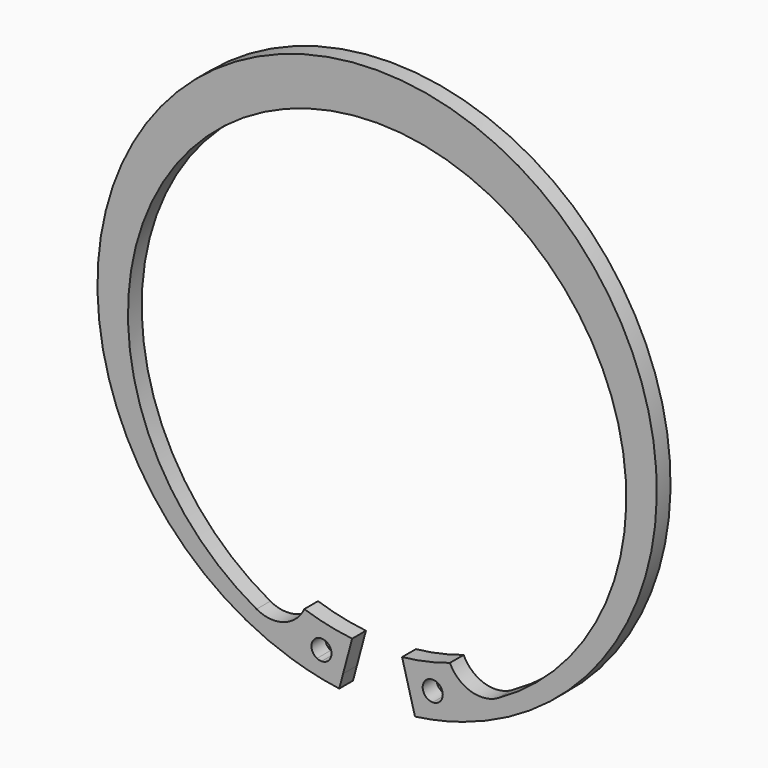
from build123d import *

# Parameters (mm, degrees)
F1_DEPTH    = 3
F2_T1_DEPTH = 3


# Not quite as in the source:
# - a fillet or chamfer that OpenCascade refuses, or shapes differently, is made with other operations: its cross-section is extruded or revolved along the edge and cut away or added


with BuildPart() as f1:
    # F0 (on Front) → F1 (new body)
    with BuildSketch(Plane.XZ):
        with BuildLine():
            Line((-12.6923788449, -38.0739606037), (-14.2292520278, -43.8096494069))
            ThreePointArc((-14.2292520278, -43.8096494069), (-12.3693152355, -44.4080485447), (-10.4843489922, -44.9221970263))
            ThreePointArc((-10.4843489922, -44.9221970263), (-10.6097140662, -41.870019803), (-7.9435705793, -43.3610533745))
            ThreePointArc((-7.9435705793, -43.3610533745), (-8.4561337122, -44.5984902415), (-9.6935705793, -45.1110533745))
            ThreePointArc((-9.6935705793, -45.1110533745), (-7.8201224186, -45.4967770693), (-5.9315086401, -45.7996446565))
            Line((-5.9315086401, -45.7996446565), (-4.35, -39.8973740589))
            ThreePointArc((-4.35, -39.8973740589), (-8.5698237047, -39.2081761686), (-12.6923788449, -38.0739606037))
        make_face()
        with BuildLine():
            Line((-14.2292520278, -43.8096494069), (-14.9257175554, -46.4088941417))
            ThreePointArc((-14.9257175554, -46.4088941417), (-10.8052141087, -47.537457316), (-6.6017256924, -48.3009287476))
            Line((-6.6017256924, -48.3009287476), (-5.9315086401, -45.7996446565))
            ThreePointArc((-5.9315086401, -45.7996446565), (-7.8201224186, -45.4967770693), (-9.6935705793, -45.1110533745))
            ThreePointArc((-9.6935705793, -45.1110533745), (-10.1000792565, -45.063184596), (-10.4843489922, -44.9221970263))
            ThreePointArc((-10.4843489922, -44.9221970263), (-12.3693152355, -44.4080485447), (-14.2292520278, -43.8096494069))
        make_face()
        with BuildLine():
            ThreePointArc((14.9257175554, -46.4088941417), (39.3966447228, -28.7135313848), (48.75, 0))
            ThreePointArc((48.75, 0), (-28.7135313848, 39.3966447228), (-14.9257175554, -46.4088941417))
            Line((-14.9257175554, -46.4088941417), (-14.2292520278, -43.8096494069))
            ThreePointArc((-14.2292520278, -43.8096494069), (-25.1843873236, 32.6155595225), (43.434381424, -2.7721802304))
            ThreePointArc((43.434381424, -2.7721802304), (35.3877397529, -27.956567554), (14.2292520278, -43.8096494069))
            Line((14.2292520278, -43.8096494069), (14.9257175554, -46.4088941417))
        make_face()
        with BuildLine():
            ThreePointArc((10.4843489922, -44.9221970263), (12.3693152355, -44.4080485447), (14.2292520278, -43.8096494069))
            Line((14.2292520278, -43.8096494069), (12.6923788449, -38.0739606037))
            ThreePointArc((12.6923788449, -38.0739606037), (8.5698237047, -39.2081761686), (4.35, -39.8973740589))
            Line((4.35, -39.8973740589), (5.9315086401, -45.7996446565))
            ThreePointArc((5.9315086401, -45.7996446565), (7.8201224186, -45.4967770693), (9.6935705793, -45.1110533745))
            ThreePointArc((9.6935705793, -45.1110533745), (8.4561337122, -42.1236165074), (11.4435705793, -43.3610533745))
            ThreePointArc((11.4435705793, -43.3610533745), (11.1846041508, -44.2771968614), (10.4843489922, -44.9221970263))
        make_face()
        with BuildLine():
            ThreePointArc((6.6017256924, -48.3009287476), (10.8052141087, -47.537457316), (14.9257175554, -46.4088941417))
            Line((14.9257175554, -46.4088941417), (14.2292520278, -43.8096494069))
            ThreePointArc((14.2292520278, -43.8096494069), (12.3693152355, -44.4080485447), (10.4843489922, -44.9221970263))
            ThreePointArc((10.4843489922, -44.9221970263), (10.1000792565, -45.063184596), (9.6935705793, -45.1110533745))
            ThreePointArc((9.6935705793, -45.1110533745), (7.8201224186, -45.4967770693), (5.9315086401, -45.7996446565))
            Line((5.9315086401, -45.7996446565), (6.6017256924, -48.3009287476))
        make_face()
    extrude(amount=F1_DEPTH)

    # F2: fillet of radius 5.9832263303 on 2 edges, made by hand

    # F2_s2 → F2_t1 (join)
    with BuildSketch(Plane.XZ):
        with BuildLine():
            ThreePointArc((21.0114203914, -40.7862000497), (16.2624097338, -41.2381768967), (12.6923788449, -38.0739606037))
            Line((12.6923788449, -38.0739606037), (12.5838858344, -38.124446895))
            ThreePointArc((12.5838858344, -38.124446895), (13.3452283796, -40.9727764638), (14.113664971, -43.8406208654))
            Line((14.113664971, -43.8406208654), (14.2684545363, -43.9227102855))
            ThreePointArc((14.2684545363, -43.9227102855), (17.7337895054, -42.5524219145), (21.0693082118, -40.8909311299))
            Line((21.0693082118, -40.8909311299), (21.0114203914, -40.7862000497))
        make_face()
        with BuildLine():
            ThreePointArc((-12.6923788449, -38.0739606037), (-16.2624097338, -41.2381768967), (-21.0114203914, -40.7862000497))
            Line((-21.0114203914, -40.7862000497), (-21.0693082118, -40.8909311299))
            ThreePointArc((-21.0693082118, -40.8909311299), (-17.7337895054, -42.5524219145), (-14.2684545363, -43.9227102855))
            Line((-14.2684545363, -43.9227102855), (-14.113664971, -43.8406208654))
            ThreePointArc((-14.113664971, -43.8406208654), (-13.3452283796, -40.9727764638), (-12.5838858345, -38.124446895))
            Line((-12.5838858345, -38.124446895), (-12.6923788449, -38.0739606037))
        make_face()
    extrude(amount=F2_T1_DEPTH)


solid = f1.part
